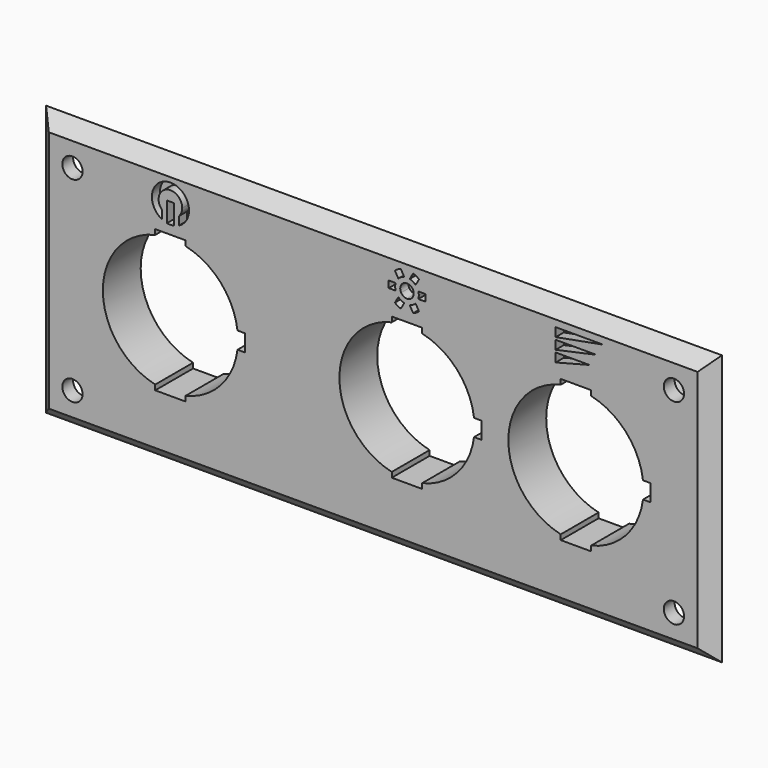
from build123d import *

# Parameters (mm, degrees)
F0_W      = 100
F0_H      = 40
F1_DEPTH  = 2
F2_SIZE   = 1.99999
F3_W      = 84
F3_H      = 24
F4_DEPTH  = 5
F5_R      = 1.5
F6_DEPTH  = 2.001
F7_R      = 5
F8_R      = 10
F9_DEPTH  = 7.001
F11_DEPTH = 7.001
F13_DEPTH = 7.001
F15_DEPTH = 1.5
F17_DEPTH = 1.5
F19_DEPTH = 1.5


# Not quite as in the source:
# - a fillet or chamfer is up to 0.001 mm smaller than in the source, because OpenCascade refuses the exact size


with BuildPart() as f1:
    # F0 (on Front) → F1 (new body)
    with BuildSketch(Plane.XZ):
        with Locations((50, 20)):
            Rectangle(F0_W, F0_H)
    extrude(amount=F1_DEPTH)

    # F2 (size 2 in the source; OpenCascade refuses exactly that, so slightly less here)
    f2_edges = [f1.edges().sort_by_distance(p)[0] for p in [
        (100, -2, 20),
        (50, -2, 40),
        (50, -2, 0),
        (0, -2, 20),
    ]]
    chamfer(f2_edges, length=F2_SIZE)

    # F3 (on face) → F4 (join)
    with BuildSketch(Plane(origin=(0, 0, 0), x_dir=(-1, 0, 0), z_dir=(0, 1, 0))):
        with Locations((-50, 20)):
            Rectangle(F3_W, F3_H)
    extrude(amount=F4_DEPTH)

    # F5 (on face) → F6 (cut, through all)
    with BuildSketch(Plane(origin=(0, 0, 0), x_dir=(-1, 0, 0), z_dir=(0, 1, 0))):
        with Locations((-94.5, 34.5)):
            Circle(F5_R)
        with Locations((-94.5, 5.5)):
            Circle(F5_R)
        with Locations((-5.5, 34.5)):
            Circle(F5_R)
        with Locations((-5.5, 5.5)):
            Circle(F5_R)
    extrude(amount=-F6_DEPTH, mode=Mode.SUBTRACT)

    # F7
    f7_edges = [f1.edges().sort_by_distance(p)[0] for p in [
        (92, 2.5, 8),
        (92, 2.5, 32),
        (8, 2.5, 8),
        (8, 2.5, 32),
    ]]
    fillet(f7_edges, radius=F7_R)

    # F8 (on face) → F9 (cut, through all)
    with BuildSketch(Plane(origin=(0, 5, 0), x_dir=(-1, 0, 0), z_dir=(0, 1, 0))):
        with Locations((-80, 20)):
            Circle(F8_R)
        with Locations((-55, 20)):
            Circle(F8_R)
        with Locations((-20, 20)):
            Circle(F8_R)
    extrude(amount=-F9_DEPTH, mode=Mode.SUBTRACT)

    # F10 (on face) → F11 (cut, through all)
    with BuildSketch(Plane(origin=(0, 5, 0), x_dir=(-1, 0, 0), z_dir=(0, 1, 0))):
        with BuildLine():
            Line((-89.9215674165, 21.25), (-91, 21.25))
            Line((-91, 21.25), (-91, 18.75))
            Line((-91, 18.75), (-89.9215674165, 18.75))
            ThreePointArc((-89.9215674165, 18.75), (-90, 20), (-89.9215674165, 21.25))
        make_face()
        with BuildLine():
            Line((-64.9215674165, 21.25), (-66, 21.25))
            Line((-66, 21.25), (-66, 18.75))
            Line((-66, 18.75), (-64.9215674165, 18.75))
            ThreePointArc((-64.9215674165, 18.75), (-65, 20), (-64.9215674165, 21.25))
        make_face()
        with BuildLine():
            Line((-29.9215674165, 21.25), (-31, 21.25))
            Line((-31, 21.25), (-31, 18.75))
            Line((-31, 18.75), (-29.9215674165, 18.75))
            ThreePointArc((-29.9215674165, 18.75), (-30, 20), (-29.9215674165, 21.25))
        make_face()
    extrude(amount=-F11_DEPTH, mode=Mode.SUBTRACT)

    # F12 (on face) → F13 (cut, through all)
    with BuildSketch(Plane(origin=(0, 5, 0), x_dir=(-1, 0, 0), z_dir=(0, 1, 0))):
        with BuildLine():
            Line((-77.75, 30.5), (-82.25, 30.5))
            Line((-82.25, 30.5), (-82.25, 29.743587635))
            ThreePointArc((-82.25, 29.743587635), (-80, 30), (-77.75, 29.743587635))
            Line((-77.75, 29.743587635), (-77.75, 30.5))
        make_face()
        with BuildLine():
            ThreePointArc((-77.75, 10.256412365), (-80, 10), (-82.25, 10.256412365))
            Line((-82.25, 10.256412365), (-82.25, 9.5))
            Line((-82.25, 9.5), (-77.75, 9.5))
            Line((-77.75, 9.5), (-77.75, 10.256412365))
        make_face()
        with BuildLine():
            ThreePointArc((-52.75, 10.256412365), (-55, 10), (-57.25, 10.256412365))
            Line((-57.25, 10.256412365), (-57.25, 9.5))
            Line((-57.25, 9.5), (-52.75, 9.5))
            Line((-52.75, 9.5), (-52.75, 10.256412365))
        make_face()
        with BuildLine():
            Line((-52.75, 30.5), (-57.25, 30.5))
            Line((-57.25, 30.5), (-57.25, 29.743587635))
            ThreePointArc((-57.25, 29.743587635), (-55, 30), (-52.75, 29.743587635))
            Line((-52.75, 29.743587635), (-52.75, 30.5))
        make_face()
        with BuildLine():
            Line((-17.75, 30.5), (-22.25, 30.5))
            Line((-22.25, 30.5), (-22.25, 29.743587635))
            ThreePointArc((-22.25, 29.743587635), (-20, 30), (-17.75, 29.743587635))
            Line((-17.75, 29.743587635), (-17.75, 30.5))
        make_face()
        with BuildLine():
            ThreePointArc((-17.75, 10.256412365), (-20, 10), (-22.25, 10.256412365))
            Line((-22.25, 10.256412365), (-22.25, 9.5))
            Line((-22.25, 9.5), (-17.75, 9.5))
            Line((-17.75, 9.5), (-17.75, 10.256412365))
        make_face()
    extrude(amount=-F13_DEPTH, mode=Mode.SUBTRACT)

    # F14 (on face) → F15 (cut)
    with BuildSketch(Plane.XZ.offset(2)):
        with BuildLine():
            ThreePointArc((22.75, 34.55), (18.5638593384, 36.8952078799), (18.75, 32.1005102572))
            Line((18.75, 32.1005102572), (18.75, 33.3252551286))
            ThreePointArc((18.75, 33.3252551286), (19.3385621722, 36.1701851746), (21.75, 34.55))
            ThreePointArc((21.75, 34.55), (21.6201851746, 33.8885621722), (21.25, 33.3252551286))
            Line((21.25, 33.3252551286), (21.25, 32.1005102572))
            ThreePointArc((21.25, 32.1005102572), (22.3452078799, 33.1138593384), (22.75, 34.55))
        make_face()
        with BuildLine():
            Line((19.5, 34.8), (19.5, 32.8729490169))
            ThreePointArc((19.5, 32.8729490169), (20, 32.8), (20.5, 32.8729490169))
            Line((20.5, 32.8729490169), (20.5, 34.8))
            Line((20.5, 34.8), (19.5, 34.8))
        make_face()
        with BuildLine():
            ThreePointArc((19.5, 31.8458365434), (19.7489517035, 31.8114831107), (20, 31.8))
            ThreePointArc((20, 31.8), (20.2510482965, 31.8114831107), (20.5, 31.8458365434))
            Line((20.5, 31.8458365434), (20.5, 32.8729490169))
            ThreePointArc((20.5, 32.8729490169), (20, 32.8), (19.5, 32.8729490169))
            Line((19.5, 32.8729490169), (19.5, 31.8458365434))
        make_face()
    extrude(amount=-F15_DEPTH, mode=Mode.SUBTRACT)

    # F16 (on face) → F17 (cut)
    with BuildSketch(Plane.XZ.offset(2)):
        with BuildLine():
            ThreePointArc((54.1339745962, 34.05), (54.5, 33.6839745962), (55, 33.55))
            Line((55, 33.55), (54.7113248654, 34.05))
            Line((54.7113248654, 34.05), (54.1339745962, 34.05))
        make_face()
        Polygon((54.4226497308, 34.55), (54.1339745962, 34.05), (54.7113248654, 34.05), align=None)
        with BuildLine():
            Line((54.4226497308, 34.55), (54.1339745962, 35.05))
            ThreePointArc((54.1339745962, 35.05), (54, 34.55), (54.1339745962, 34.05))
            Line((54.1339745962, 34.05), (54.4226497308, 34.55))
        make_face()
        Polygon((54.7113248654, 35.05), (54.1339745962, 35.05), (54.4226497308, 34.55), align=None)
        with BuildLine():
            Line((54.7113248654, 35.05), (55, 35.55))
            ThreePointArc((55, 35.55), (54.5, 35.4160254038), (54.1339745962, 35.05))
            Line((54.1339745962, 35.05), (54.7113248654, 35.05))
        make_face()
        Polygon((55.2886751346, 35.05), (55, 35.55), (54.7113248654, 35.05), align=None)
        Polygon((55.5773502692, 34.55), (55.2886751346, 35.05), (54.7113248654, 35.05), (54.4226497308, 34.55), (54.7113248654, 34.05), (55.2886751346, 34.05), align=None)
        Polygon((54.7113248654, 34.05), (55, 33.55), (55.2886751346, 34.05), align=None)
        with BuildLine():
            ThreePointArc((55, 33.55), (55.5, 33.6839745962), (55.8660254038, 34.05))
            Line((55.8660254038, 34.05), (55.2886751346, 34.05))
            Line((55.2886751346, 34.05), (55, 33.55))
        make_face()
        with BuildLine():
            ThreePointArc((56, 34.55), (55.9659258263, 34.8088190451), (55.8660254038, 35.05))
            Line((55.8660254038, 35.05), (55.5773502692, 34.55))
            Line((55.5773502692, 34.55), (55.8660254038, 34.05))
            ThreePointArc((55.8660254038, 34.05), (55.9659258263, 34.2911809549), (56, 34.55))
        make_face()
        Polygon((55.5773502692, 34.55), (55.8660254038, 35.05), (55.2886751346, 35.05), align=None)
        with BuildLine():
            Line((55.2886751346, 35.05), (55.8660254038, 35.05))
            ThreePointArc((55.8660254038, 35.05), (55.5, 35.4160254038), (55, 35.55))
            Line((55, 35.55), (55.2886751346, 35.05))
        make_face()
        Polygon((55.2886751346, 34.05), (55.8660254038, 34.05), (55.5773502692, 34.55), align=None)
        with BuildLine():
            ThreePointArc((53.2149055698, 32.4581257506), (53.625, 32.1684301396), (54.0809309736, 31.9581257506))
            Line((54.0809309736, 31.9581257506), (54.5944872103, 32.8476312452))
            ThreePointArc((54.5944872103, 32.8476312452), (54.125, 33.0344555434), (53.7284618065, 33.3476312452))
            Line((53.7284618065, 33.3476312452), (53.2149055698, 32.4581257506))
        make_face()
        with BuildLine():
            ThreePointArc((55.9190690264, 31.9581257506), (56.375, 32.1684301396), (56.7850944302, 32.4581257506))
            Line((56.7850944302, 32.4581257506), (56.2715381935, 33.3476312452))
            ThreePointArc((56.2715381935, 33.3476312452), (55.875, 33.0344555434), (55.4055127897, 32.8476312452))
            Line((55.4055127897, 32.8476312452), (55.9190690264, 31.9581257506))
        make_face()
        with BuildLine():
            ThreePointArc((57.7041634566, 34.05), (57.7385168893, 34.2989517035), (57.75, 34.55))
            ThreePointArc((57.75, 34.55), (57.7385168893, 34.8010482965), (57.7041634566, 35.05))
            Line((57.7041634566, 35.05), (56.6770509831, 35.05))
            ThreePointArc((56.6770509831, 35.05), (56.7316667145, 34.8026467688), (56.75, 34.55))
            ThreePointArc((56.75, 34.55), (56.7316667145, 34.2973532312), (56.6770509831, 34.05))
            Line((56.6770509831, 34.05), (57.7041634566, 34.05))
        make_face()
        with BuildLine():
            Line((56.2715381935, 35.7523687548), (56.7850944302, 36.6418742494))
            ThreePointArc((56.7850944302, 36.6418742494), (56.375, 36.9315698604), (55.9190690264, 37.1418742494))
            Line((55.9190690264, 37.1418742494), (55.4055127897, 36.2523687548))
            ThreePointArc((55.4055127897, 36.2523687548), (55.875, 36.0655444566), (56.2715381935, 35.7523687548))
        make_face()
        with BuildLine():
            Line((54.5944872103, 36.2523687548), (54.0809309736, 37.1418742494))
            ThreePointArc((54.0809309736, 37.1418742494), (53.625, 36.9315698604), (53.2149055698, 36.6418742494))
            Line((53.2149055698, 36.6418742494), (53.7284618065, 35.7523687548))
            ThreePointArc((53.7284618065, 35.7523687548), (54.125, 36.0655444566), (54.5944872103, 36.2523687548))
        make_face()
        with BuildLine():
            Line((53.3229490169, 35.05), (52.2958365434, 35.05))
            ThreePointArc((52.2958365434, 35.05), (52.25, 34.55), (52.2958365434, 34.05))
            Line((52.2958365434, 34.05), (53.3229490169, 34.05))
            ThreePointArc((53.3229490169, 34.05), (53.25, 34.55), (53.3229490169, 35.05))
        make_face()
    extrude(amount=-F17_DEPTH, mode=Mode.SUBTRACT)

    # F18 (on face) → F19 (cut)
    with BuildSketch(Plane.XZ.offset(2)):
        Polygon((77, 35.7), (84, 37), (77, 37), align=None)
        Polygon((83, 35.35), (77, 35.35), (77, 34.05), align=None)
        Polygon((77, 32.4), (82, 33.7), (77, 33.7), align=None)
    extrude(amount=-F19_DEPTH, mode=Mode.SUBTRACT)


solid = f1.part
